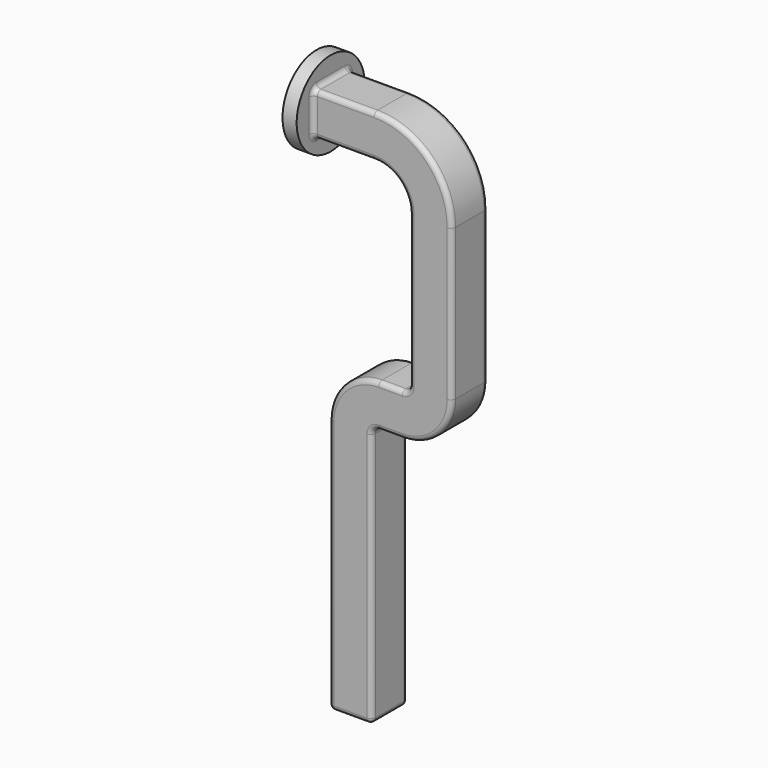
from build123d import *

# Parameters (mm, degrees)
F0_R     = 45
F1_DEPTH = 15
F2_W     = 47.7026963846
F2_H     = 45
F5_F1_R  = 5
F5_F2_R  = 5


with BuildPart() as f1:
    # F0 (on Right) → F1 (new body)
    with BuildSketch(Plane.YZ):
        Circle(F0_R)
    extrude(amount=F1_DEPTH)

    # F4: sweep along a path in F3
    with BuildLine(Plane.XZ) as f4_path:
        Line((15, 0), (80, 0))
        ThreePointArc((80, 0), (122.4264068712, -17.5735931288), (140, -60))
        Line((140, -60), (140, -220))
        ThreePointArc((140, -220), (131.2132034356, -241.2132034356), (110, -250))
        Line((110, -250), (85, -250))
        ThreePointArc((85, -250), (63.7867965644, -258.7867965644), (55, -280))
        Line((55, -280), (55, -550))
    # F2 (on face) → F4 (sweep)
    with BuildSketch(Plane.YZ.offset(15)):
        Rectangle(F2_W, F2_H)
    sweep(path=f4_path.line)

    # F5: fillet of radius 5 on 34 edges, made by hand

    # F5_f1
    f5_f1_edges = [f1.edges().sort_by_distance(p)[0] for p in [
        (47.5, -23.8513481923, 22.5),
        (47.5, -23.8513481923, -22.5),
        (106.5165042945, -23.8513481923, -33.4834957055),
        (117.5, -23.8513481923, -140),
        (115.3033008589, -23.8513481923, -225.3033008589),
        (97.5, -23.8513481923, -227.5),
        (47.8768939877, -23.8513481923, -242.8768939877),
        (32.5, -23.8513481923, -415),
        (55, -23.8513481923, -550),
        (77.5, -23.8513481923, -415),
        (79.6966991411, -23.8513481923, -274.6966991411),
        (97.5, -23.8513481923, -272.5),
        (147.1231060123, -23.8513481923, -257.1231060123),
        (162.5, -23.8513481923, -140),
        (138.3363094479, -23.8513481923, -1.6636905521),
        (47.5, 23.8513481923, -22.5),
        (47.5, 23.8513481923, 22.5),
        (138.3363094479, 23.8513481923, -1.6636905521),
        (162.5, 23.8513481923, -140),
        (147.1231060123, 23.8513481923, -257.1231060123),
        (97.5, 23.8513481923, -272.5),
        (79.6966991411, 23.8513481923, -274.6966991411),
        (77.5, 23.8513481923, -415),
        (55, 23.8513481923, -550),
        (32.5, 23.8513481923, -415),
        (47.8768939877, 23.8513481923, -242.8768939877),
        (97.5, 23.8513481923, -227.5),
        (115.3033008589, 23.8513481923, -225.3033008589),
        (117.5, 23.8513481923, -140),
        (106.5165042945, 23.8513481923, -33.4834957055),
        (32.5, 0, -550),
        (77.5, 0, -550),
    ]]
    fillet(f5_f1_edges, radius=F5_F1_R)

    # F5_f2
    f5_f2_edges = [f1.edges().sort_by_distance(p)[0] for p in [
        (15, -23.8513481923, 0),
        (15, 23.8513481923, 0),
        (15, 22.3868820983, -21.0355339059),
        (15, 22.3868820983, 21.0355339059),
        (15, -22.3868820983, 21.0355339059),
        (15, -22.3868820983, -21.0355339059),
    ]]
    fillet(f5_f2_edges, radius=F5_F2_R)


solid = f1.part
